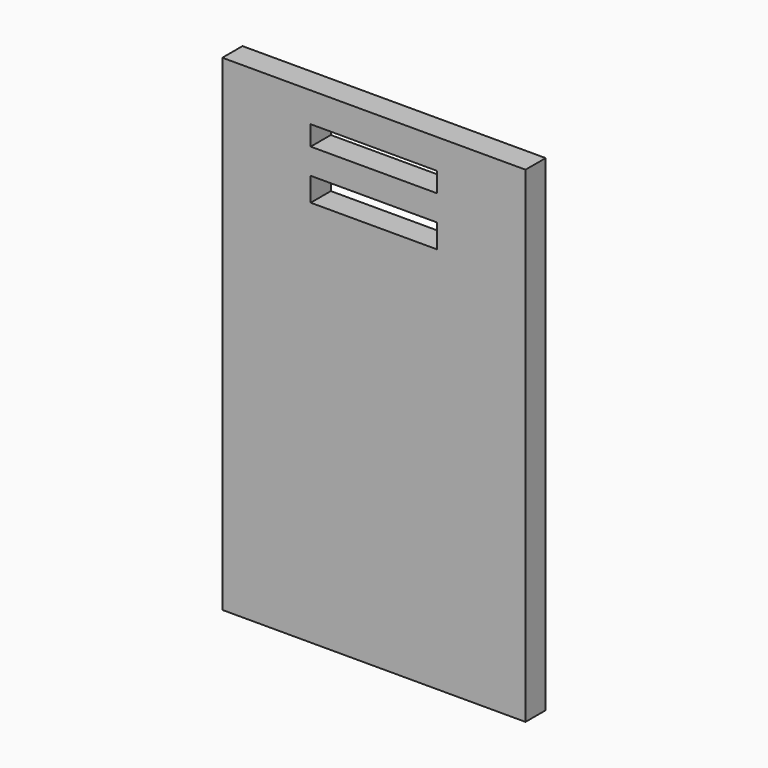
from build123d import *

# Parameters (mm, degrees)
F0_W           = 305.8499656135
F0_H           = 490.4834032059
F0_W_2         = 127.6116371155
F0_H_2         = 23.9074826241
F0_H_3         = 19.9229419231
F1_DEPTH       = 25.4
F2_TEXT_SIZE   = 42.8896293872
F3_DEPTH       = 7.62
F4_R           = 60.5262004627
F5_DEPTH       = 7.62
F6_R           = 52.1002280799
F7_DEPTH       = 7.62
F8_TEXT_SIZE   = 20.0911295704
F8_TEXT_SIZE_2 = 21.9175947778
F8_TEXT_SIZE_3 = 21.9175928376
F8_TEXT_SIZE_4 = 21.0043605572
F9_DEPTH       = 5.08


# Not quite as in the source:
# - Text() gives the source's letters only with a copy of the font that has no kerning and outlines rounded to 1/6400 em; it was checked with that copy


with BuildPart() as f1:
    # F0 (on Front) → F1 (new body)
    with BuildSketch(Plane.XZ):
        Rectangle(F0_W, F0_H)
        with Locations((0, 157.3911011219)):
            Rectangle(F0_W_2, F0_H_2, mode=Mode.SUBTRACT)
        with Locations((0, 205.2061110735)):
            Rectangle(F0_W_2, F0_H_3, mode=Mode.SUBTRACT)
    extrude(amount=F1_DEPTH)

    # F2 (on face) → F3 (join)
    with BuildSketch(Plane(origin=(0, 0, 0), x_dir=(-1, 0, 0), z_dir=(0, 1, 0))):
        with Locations((-35.9137263149, 86.6647064686)):
            Text('999', F2_TEXT_SIZE, font='Open Sans', text_align=(TextAlign.LEFT, TextAlign.BOTTOM))
    extrude(amount=F3_DEPTH)

    # F4 (on face) → F5 (join)
    with BuildSketch(Plane(origin=(0, 0, 0), x_dir=(-1, 0, 0), z_dir=(0, 1, 0))):
        Circle(F4_R)
    extrude(amount=F5_DEPTH)

    # F6 (on face) → F7 (join)
    with BuildSketch(Plane(origin=(0, 7.62, 0), x_dir=(-1, 0, 0), z_dir=(0, 1, 0))):
        Circle(F6_R)
    extrude(amount=F7_DEPTH)

    # F8 (on face) → F9 (join)
    with BuildSketch(Plane(origin=(0, 15.24, 0), x_dir=(-1, 0, 0), z_dir=(0, 1, 0))):
        with Locations((-13.0312610418, 31.6880363971)):
            Text('10', F8_TEXT_SIZE, font='Open Sans', text_align=(TextAlign.LEFT, TextAlign.BOTTOM))
        with Locations((22.4752351642, -8.7499220972)):
            Text('30', F8_TEXT_SIZE_2, font='Open Sans', text_align=(TextAlign.LEFT, TextAlign.BOTTOM))
        with Locations((-10.40115254, -46.2290067226)):
            Text('60', F8_TEXT_SIZE_3, font='Open Sans', text_align=(TextAlign.LEFT, TextAlign.BOTTOM))
        with Locations((-46.5651862323, -8.7499213405)):
            Text('90', F8_TEXT_SIZE_4, font='Open Sans', text_align=(TextAlign.LEFT, TextAlign.BOTTOM))
    extrude(amount=F9_DEPTH)


solid = f1.part
